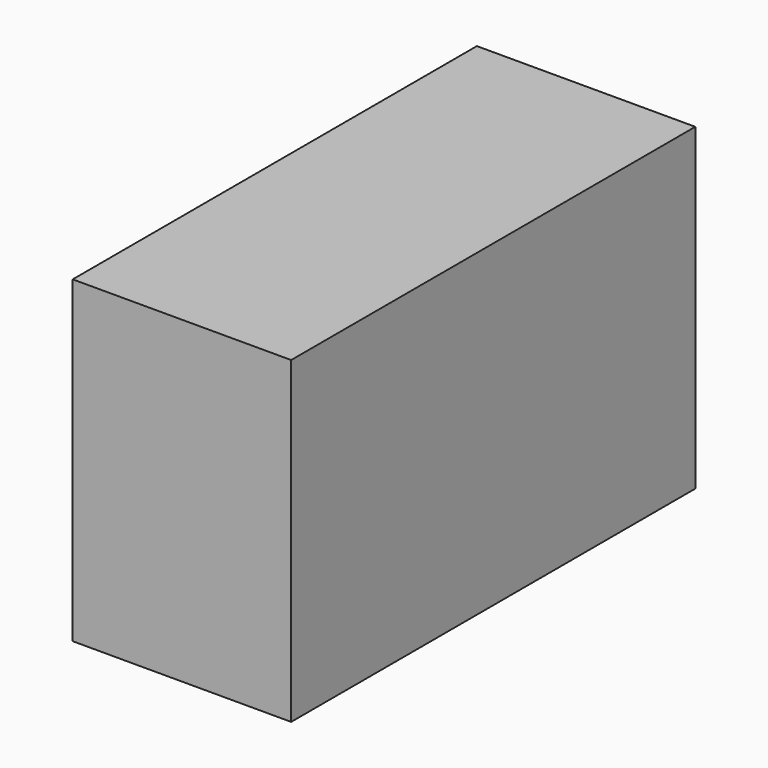
from build123d import *

# Parameters (mm, degrees)
F0_W     = 480
F0_H     = 1110
F1_DEPTH = 350
F2_T     = -10


# Not quite as in the source:
# - the program builds the solid bodies; features that only make, move or delete a surface that nothing else refers to are left out


with BuildPart() as f1:
    # F0 (on Top) → F1 (new body, symmetric)
    with BuildSketch(Plane.XY):
        Rectangle(F0_W, F0_H)
    extrude(amount=F1_DEPTH, both=True)

    # F2 (hollow: no face is removed)
    offset(amount=F2_T, mode=Mode.SUBTRACT)


solid = f1.part
